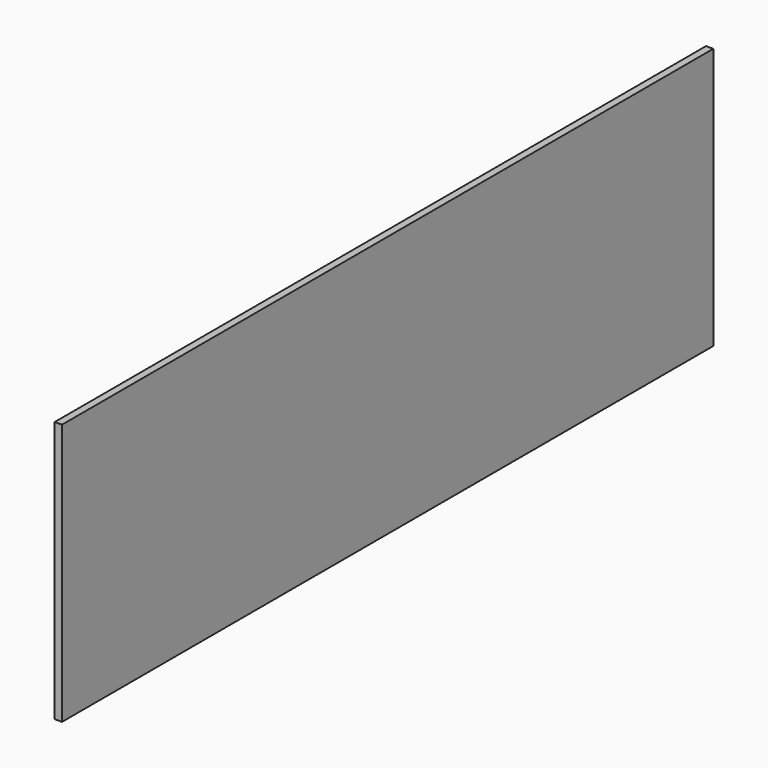
from build123d import *

# Parameters (mm, degrees)
F0_W     = 533.4
F0_H     = 171.45
F1_DEPTH = 4.7625


# Not quite as in the source:
# - a length typed as a fraction of an inch, garbled in the dataset ("3 / 203.2 mm" for 3/8 in), is restored


with BuildPart() as f1:
    # F0 (on Right) → F1 (new body)
    with BuildSketch(Plane.YZ):
        with Locations((-101.5250182853, -358.5250534113)):
            Rectangle(F0_W, F0_H)
    extrude(amount=-F1_DEPTH)


solid = f1.part
